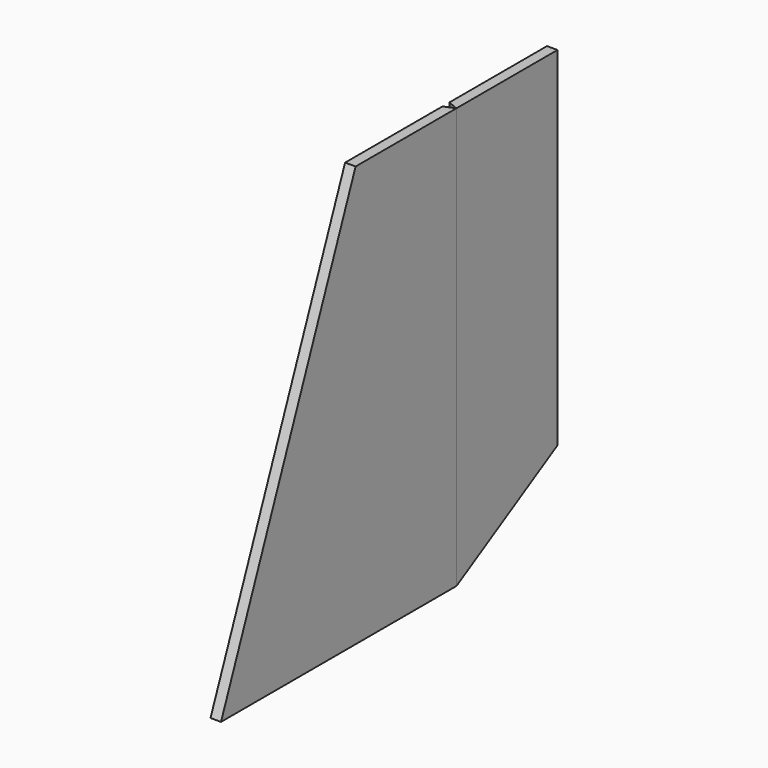
from build123d import *

# Parameters (mm, degrees)
F1_DEPTH    = 1.5875
F2_DEPTH    = 1.5875
F3_T1_DEPTH = 144.1219952748
F4_SIZE2    = 1.2625229381
F4_SIZE     = 3.048


# Not quite as in the source:
# - a fillet or chamfer that OpenCascade refuses, or shapes differently, is made with other operations: its cross-section is extruded or revolved along the edge and cut away or added


with BuildPart() as f1:
    # F0 (on Right) → F1 (new body, symmetric)
    with BuildSketch(Plane.YZ):
        Polygon((-88.9, 0), (0, 0), (0, 127), (-38.1, 127), align=None)
    extrude(amount=F1_DEPTH, both=True)

    # F3: chamfer of 3.302 x 1.367733183 on 1 edges, made by hand

    # F3_s2 → F3_t1 (cut)
    with BuildSketch(Plane.XY.offset(-8.5609976374)):
        Polygon((1.7145, 0), (-1.5875, -1.367733183), (-1.5875, 0), align=None)
    extrude(amount=F3_T1_DEPTH, mode=Mode.SUBTRACT)


with BuildPart() as f2:
    # F0 (on Right) → F2 (new body, symmetric)
    with BuildSketch(Plane.YZ):
        Polygon((0, 127), (0, 0), (38.1, 21.900890395), (38.1, 127), align=None)
    extrude(amount=F2_DEPTH, both=True)

    # F4
    f4_edges = [f2.edges().sort_by_distance(p)[0] for p in [
        (-1.5875, 0, 63.5),
    ]]
    f4_side = f2.faces().sort_by_distance((0, 0, 63.5))[0]
    chamfer(f4_edges, length=F4_SIZE, length2=F4_SIZE2, reference=f4_side)


solid = Compound([f1.part, f2.part])
